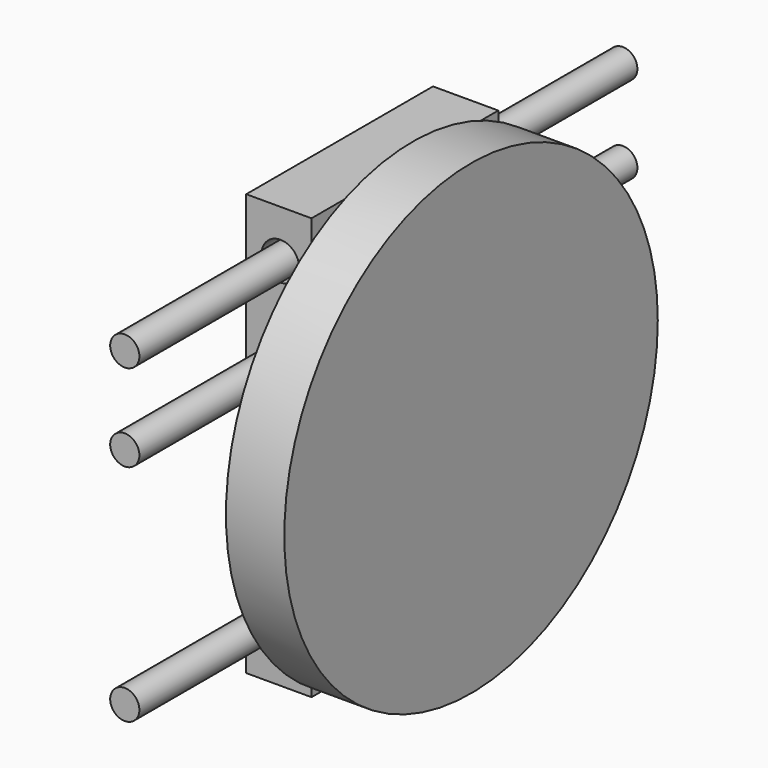
from build123d import *

# Parameters (mm, degrees)
F0_R     = 4.7625
F1_DEPTH = 101.6
F2_R     = 76.2
F2_R_2   = 9.525
F3_DEPTH = 19.05
F4_DEPTH = 50.8
F5_W     = 21.3117243114
F5_H     = 137.6228183508
F5_R     = 5.7912992377
F5_R_2   = 6.0348069949
F5_R_3   = 6.155398866
F6_DEPTH = 38.1
F7_R     = 9.9788565771
F8_DEPTH = 42.9027243114


with BuildPart() as f1:
    # F0 (on Front) → F1 (new body, symmetric)
    with BuildSketch(Plane.XZ):
        with Locations((-31.75, 53.2060163036)):
            Circle(F0_R)
    extrude(amount=F1_DEPTH, both=True)


with BuildPart() as f1b:
    # F0 (on Front) → F1, piece 2 (new body, symmetric)
    with BuildSketch(Plane.XZ):
        with Locations((-31.75, -48.3939836964)):
            Circle(F0_R)
    extrude(amount=F1_DEPTH, both=True)


with BuildPart() as f1c:
    # F0 (on Front) → F1, piece 3 (new body, symmetric)
    with BuildSketch(Plane.XZ):
        with Locations((-31.75, 24.7723255306)):
            Circle(F0_R)
    extrude(amount=F1_DEPTH, both=True)


with BuildPart() as f3:
    # F2 (on Right) → F3 (new body)
    with BuildSketch(Plane.YZ):
        Circle(F2_R)
        Circle(F2_R_2, mode=Mode.SUBTRACT)
    extrude(amount=-F3_DEPTH)

    # F2 (on Right) → F4 (join)
    with BuildSketch(Plane.YZ):
        Circle(F2_R_2)
    extrude(amount=-F4_DEPTH)


with BuildPart() as f6:
    # F5 (on Front) → F6 (new body, symmetric)
    with BuildSketch(Plane.XZ):
        with Locations((-32.2458621557, 0)):
            Rectangle(F5_W, F5_H)
        with Locations((-31.75, -48.3939836964)):
            Circle(F5_R, mode=Mode.SUBTRACT)
        with Locations((-31.75, 24.7723255306)):
            Circle(F5_R_2, mode=Mode.SUBTRACT)
        with Locations((-31.75, 53.2060163036)):
            Circle(F5_R_3, mode=Mode.SUBTRACT)
    extrude(amount=F6_DEPTH, both=True)

    # F7 (on face) → F8 (cut, through all)
    with BuildSketch(Plane(origin=(-42.9017243114, 0, 0), x_dir=(0, -1, 0), z_dir=(-1, 0, 0))):
        Circle(F7_R)
    extrude(amount=-F8_DEPTH, mode=Mode.SUBTRACT)


solid = Compound([f1.part, f1b.part, f1c.part, f3.part, f6.part])
